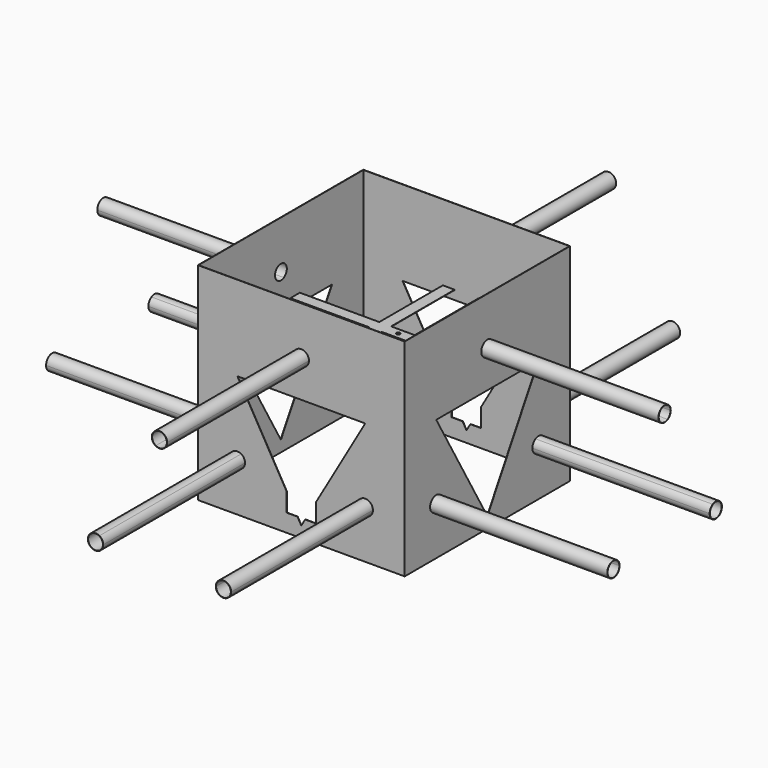
from build123d import *

# Parameters (mm, degrees)
F0_W      = 700
F0_H      = 700
F0_W_2    = 698
F0_H_2    = 698
F1_DEPTH  = 700
F6_DEPTH  = 600
F7_DEPTH  = 600
F8_DEPTH  = 600
F9_DEPTH  = 600
F10_DEPTH = 25
F11_DEPTH = 25
F12_DEPTH = 25
F13_DEPTH = 25
F14_DEPTH = 25
F15_DEPTH = 25
F16_DEPTH = 4990
F17_DEPTH = 700
F18_DEPTH = 700
F19_DEPTH = 700
F20_DEPTH = 700
F21_W     = 100
F21_H     = 80
F22_DEPTH = 350
F24_D     = 13
F24_DEPTH = 5
F24_TIP   = 3.905594


with BuildPart() as f1:
    # F0 (on Top) → F1 (new body)
    with BuildSketch(Plane.XY):
        Rectangle(F0_W, F0_H)
        Rectangle(F0_W_2, F0_H_2, mode=Mode.SUBTRACT)
    extrude(amount=-F1_DEPTH)

    # F2 (on face) → F6 (join)
    with BuildSketch(Plane.YZ.offset(350)):
        with BuildLine():
            ThreePointArc((25, -162.5), (21.650635, -175), (12.5, -184.150635))
            Line((12.5, -184.150635), (13, -185.01666))
            ThreePointArc((13, -185.01666), (22.51666, -175.5), (26, -162.5))
            ThreePointArc((26, -162.5), (-13, -139.98334), (-13, -185.01666))
            Line((-13, -185.01666), (-12.5, -184.150635))
            ThreePointArc((-12.5, -184.150635), (-12.5, -140.849365), (25, -162.5))
        make_face()
        with BuildLine():
            ThreePointArc((242.506351, -537.5), (229.506351, -514.98334), (203.506351, -514.98334))
            Line((203.506351, -514.98334), (204.006351, -515.849365))
            ThreePointArc((204.006351, -515.849365), (229.006351, -515.849365), (241.506351, -537.5))
            ThreePointArc((241.506351, -537.5), (216.506351, -562.5), (191.506351, -537.5))
            Line((191.506351, -537.5), (190.506351, -537.5))
            ThreePointArc((190.506351, -537.5), (216.506351, -563.5), (242.506351, -537.5))
        make_face()
        with BuildLine():
            Line((204.006351, -515.849365), (203.506351, -514.98334))
            ThreePointArc((203.506351, -514.98334), (193.98969, -524.5), (190.506351, -537.5))
            Line((190.506351, -537.5), (191.506351, -537.5))
            ThreePointArc((191.506351, -537.5), (194.855716, -525), (204.006351, -515.849365))
        make_face()
        with BuildLine():
            Line((13, -185.01666), (12.5, -184.150635))
            ThreePointArc((12.5, -184.150635), (0, -187.5), (-12.5, -184.150635))
            Line((-12.5, -184.150635), (-13, -185.01666))
            ThreePointArc((-13, -185.01666), (0, -188.5), (13, -185.01666))
        make_face()
        with BuildLine():
            Line((-204.006351, -515.849365), (-203.506351, -514.98334))
            ThreePointArc((-203.506351, -514.98334), (-239.023011, -550.5), (-190.506351, -537.5))
            Line((-190.506351, -537.5), (-191.506351, -537.5))
            ThreePointArc((-191.506351, -537.5), (-238.156986, -550), (-204.006351, -515.849365))
        make_face()
        with BuildLine():
            ThreePointArc((-190.506351, -537.5), (-193.98969, -524.5), (-203.506351, -514.98334))
            Line((-203.506351, -514.98334), (-204.006351, -515.849365))
            ThreePointArc((-204.006351, -515.849365), (-194.855716, -525), (-191.506351, -537.5))
            Line((-191.506351, -537.5), (-190.506351, -537.5))
        make_face()
    extrude(amount=F6_DEPTH)

    # F3 (on face) → F7 (join)
    with BuildSketch(Plane.XZ.offset(350)):
        with BuildLine():
            Line((13, -185.01666), (12.5, -184.150635))
            ThreePointArc((12.5, -184.150635), (0, -187.5), (-12.5, -184.150635))
            Line((-12.5, -184.150635), (-13, -185.01666))
            ThreePointArc((-13, -185.01666), (0, -188.5), (13, -185.01666))
        make_face()
        with BuildLine():
            ThreePointArc((25, -162.5), (21.650635, -175), (12.5, -184.150635))
            Line((12.5, -184.150635), (13, -185.01666))
            ThreePointArc((13, -185.01666), (22.51666, -175.5), (26, -162.5))
            ThreePointArc((26, -162.5), (-13, -139.98334), (-13, -185.01666))
            Line((-13, -185.01666), (-12.5, -184.150635))
            ThreePointArc((-12.5, -184.150635), (-12.5, -140.849365), (25, -162.5))
        make_face()
        with BuildLine():
            Line((-204.006351, -515.849365), (-203.506351, -514.98334))
            ThreePointArc((-203.506351, -514.98334), (-239.023011, -550.5), (-190.506351, -537.5))
            Line((-190.506351, -537.5), (-191.506351, -537.5))
            ThreePointArc((-191.506351, -537.5), (-238.156986, -550), (-204.006351, -515.849365))
        make_face()
        with BuildLine():
            ThreePointArc((-190.506351, -537.5), (-193.98969, -524.5), (-203.506351, -514.98334))
            Line((-203.506351, -514.98334), (-204.006351, -515.849365))
            ThreePointArc((-204.006351, -515.849365), (-194.855716, -525), (-191.506351, -537.5))
            Line((-191.506351, -537.5), (-190.506351, -537.5))
        make_face()
        with BuildLine():
            ThreePointArc((242.506351, -537.5), (229.506351, -514.98334), (203.506351, -514.98334))
            Line((203.506351, -514.98334), (204.006351, -515.849365))
            ThreePointArc((204.006351, -515.849365), (229.006351, -515.849365), (241.506351, -537.5))
            ThreePointArc((241.506351, -537.5), (216.506351, -562.5), (191.506351, -537.5))
            Line((191.506351, -537.5), (190.506351, -537.5))
            ThreePointArc((190.506351, -537.5), (216.506351, -563.5), (242.506351, -537.5))
        make_face()
        with BuildLine():
            Line((204.006351, -515.849365), (203.506351, -514.98334))
            ThreePointArc((203.506351, -514.98334), (193.98969, -524.5), (190.506351, -537.5))
            Line((190.506351, -537.5), (191.506351, -537.5))
            ThreePointArc((191.506351, -537.5), (194.855716, -525), (204.006351, -515.849365))
        make_face()
    extrude(amount=F7_DEPTH)

    # F4 (on face) → F8 (join)
    with BuildSketch(Plane(origin=(-350, 0, 0), x_dir=(0, -1, 0), z_dir=(-1, 0, 0))):
        with BuildLine():
            ThreePointArc((25, -162.5), (21.650635, -175), (12.5, -184.150635))
            Line((12.5, -184.150635), (13, -185.01666))
            ThreePointArc((13, -185.01666), (22.51666, -175.5), (26, -162.5))
            ThreePointArc((26, -162.5), (-13, -139.98334), (-13, -185.01666))
            Line((-13, -185.01666), (-12.5, -184.150635))
            ThreePointArc((-12.5, -184.150635), (-12.5, -140.849365), (25, -162.5))
        make_face()
        with BuildLine():
            Line((13, -185.01666), (12.5, -184.150635))
            ThreePointArc((12.5, -184.150635), (0, -187.5), (-12.5, -184.150635))
            Line((-12.5, -184.150635), (-13, -185.01666))
            ThreePointArc((-13, -185.01666), (0, -188.5), (13, -185.01666))
        make_face()
        with BuildLine():
            ThreePointArc((242.506351, -537.5), (229.506351, -514.98334), (203.506351, -514.98334))
            Line((203.506351, -514.98334), (204.006351, -515.849365))
            ThreePointArc((204.006351, -515.849365), (229.006351, -515.849365), (241.506351, -537.5))
            ThreePointArc((241.506351, -537.5), (216.506351, -562.5), (191.506351, -537.5))
            Line((191.506351, -537.5), (190.506351, -537.5))
            ThreePointArc((190.506351, -537.5), (216.506351, -563.5), (242.506351, -537.5))
        make_face()
        with BuildLine():
            Line((204.006351, -515.849365), (203.506351, -514.98334))
            ThreePointArc((203.506351, -514.98334), (193.98969, -524.5), (190.506351, -537.5))
            Line((190.506351, -537.5), (191.506351, -537.5))
            ThreePointArc((191.506351, -537.5), (194.855716, -525), (204.006351, -515.849365))
        make_face()
        with BuildLine():
            Line((-204.006351, -515.849365), (-203.506351, -514.98334))
            ThreePointArc((-203.506351, -514.98334), (-239.023011, -550.5), (-190.506351, -537.5))
            Line((-190.506351, -537.5), (-191.506351, -537.5))
            ThreePointArc((-191.506351, -537.5), (-238.156986, -550), (-204.006351, -515.849365))
        make_face()
        with BuildLine():
            ThreePointArc((-190.506351, -537.5), (-193.98969, -524.5), (-203.506351, -514.98334))
            Line((-203.506351, -514.98334), (-204.006351, -515.849365))
            ThreePointArc((-204.006351, -515.849365), (-194.855716, -525), (-191.506351, -537.5))
            Line((-191.506351, -537.5), (-190.506351, -537.5))
        make_face()
    extrude(amount=F8_DEPTH)

    # F5 (on face) → F9 (join)
    with BuildSketch(Plane(origin=(0, 350, 0), x_dir=(-1, 0, 0), z_dir=(0, 1, 0))):
        with BuildLine():
            Line((13, -185.01666), (12.5, -184.150635))
            ThreePointArc((12.5, -184.150635), (0, -187.5), (-12.5, -184.150635))
            Line((-12.5, -184.150635), (-13, -185.01666))
            ThreePointArc((-13, -185.01666), (0, -188.5), (13, -185.01666))
        make_face()
        with BuildLine():
            ThreePointArc((25, -162.5), (21.650635, -175), (12.5, -184.150635))
            Line((12.5, -184.150635), (13, -185.01666))
            ThreePointArc((13, -185.01666), (22.51666, -175.5), (26, -162.5))
            ThreePointArc((26, -162.5), (-13, -139.98334), (-13, -185.01666))
            Line((-13, -185.01666), (-12.5, -184.150635))
            ThreePointArc((-12.5, -184.150635), (-12.5, -140.849365), (25, -162.5))
        make_face()
        with BuildLine():
            Line((-204.006351, -515.849365), (-203.506351, -514.98334))
            ThreePointArc((-203.506351, -514.98334), (-239.023011, -550.5), (-190.506351, -537.5))
            Line((-190.506351, -537.5), (-191.506351, -537.5))
            ThreePointArc((-191.506351, -537.5), (-238.156986, -550), (-204.006351, -515.849365))
        make_face()
        with BuildLine():
            ThreePointArc((-190.506351, -537.5), (-193.98969, -524.5), (-203.506351, -514.98334))
            Line((-203.506351, -514.98334), (-204.006351, -515.849365))
            ThreePointArc((-204.006351, -515.849365), (-194.855716, -525), (-191.506351, -537.5))
            Line((-191.506351, -537.5), (-190.506351, -537.5))
        make_face()
        with BuildLine():
            Line((204.006351, -515.849365), (203.506351, -514.98334))
            ThreePointArc((203.506351, -514.98334), (193.98969, -524.5), (190.506351, -537.5))
            Line((190.506351, -537.5), (191.506351, -537.5))
            ThreePointArc((191.506351, -537.5), (194.855716, -525), (204.006351, -515.849365))
        make_face()
        with BuildLine():
            ThreePointArc((242.506351, -537.5), (229.506351, -514.98334), (203.506351, -514.98334))
            Line((203.506351, -514.98334), (204.006351, -515.849365))
            ThreePointArc((204.006351, -515.849365), (229.006351, -515.849365), (241.506351, -537.5))
            ThreePointArc((241.506351, -537.5), (216.506351, -562.5), (191.506351, -537.5))
            Line((191.506351, -537.5), (190.506351, -537.5))
            ThreePointArc((190.506351, -537.5), (216.506351, -563.5), (242.506351, -537.5))
        make_face()
    extrude(amount=F9_DEPTH)

    # F10 (cut): a face of the model
    f10_faces = [f1.faces().sort_by_distance(p)[0] for p in [
        (350, -216.506351, -537.5),
    ]]
    extrude(f10_faces, amount=-F10_DEPTH, mode=Mode.SUBTRACT)

    # F11 (cut): a face of the model
    f11_faces = [f1.faces().sort_by_distance(p)[0] for p in [
        (350, 216.506351, -537.5),
    ]]
    extrude(f11_faces, amount=-F11_DEPTH, mode=Mode.SUBTRACT)

    # F12 (cut): a face of the model
    f12_faces = [f1.faces().sort_by_distance(p)[0] for p in [
        (-350, 216.506351, -537.5),
    ]]
    extrude(f12_faces, amount=-F12_DEPTH, mode=Mode.SUBTRACT)

    # F13 (cut): a face of the model
    f13_faces = [f1.faces().sort_by_distance(p)[0] for p in [
        (-350, -216.506351, -537.5),
    ]]
    extrude(f13_faces, amount=-F13_DEPTH, mode=Mode.SUBTRACT)

    # F14 (cut): faces of the model
    f14_faces = [f1.faces().sort_by_distance(p)[0] for p in [
        (-216.506351, 350, -537.5),
        (216.506351, 350, -537.5),
    ]]
    extrude(f14_faces, amount=-F14_DEPTH, mode=Mode.SUBTRACT)

    # F15 (cut): faces of the model
    f15_faces = [f1.faces().sort_by_distance(p)[0] for p in [
        (216.506351, -350, -537.5),
        (-216.506351, -350, -537.5),
    ]]
    extrude(f15_faces, amount=-F15_DEPTH, mode=Mode.SUBTRACT)

    # F16 (cut): a face of the model
    f16_faces = [f1.faces().sort_by_distance(p)[0] for p in [
        (350, 0, -162.5),
    ]]
    extrude(f16_faces, amount=-F16_DEPTH, mode=Mode.SUBTRACT)

    # F2 (on face) → F17 (cut)
    with BuildSketch(Plane.YZ.offset(350)):
        Polygon((216.506351, -287.5), (72.168784, -287.5), (144.337567, -412.5), align=None)
        Polygon((144.337567, -412.5), (72.168784, -287.5), (-72.168784, -287.5), (-144.337567, -412.5), (-72.168784, -537.5), (72.168784, -537.5), align=None)
        Polygon((-144.337567, -412.5), (-72.168784, -287.5), (-216.506351, -287.5), align=None)
        Polygon((0, -662.5), (72.168784, -537.5), (-72.168784, -537.5), align=None)
    extrude(amount=-F17_DEPTH, mode=Mode.SUBTRACT)

    # F3 (on face) → F18 (cut)
    with BuildSketch(Plane.XZ.offset(350)):
        Polygon((-144.337567, -412.5), (-72.168784, -287.5), (-216.506351, -287.5), align=None)
        Polygon((144.337567, -412.5), (72.168784, -287.5), (-72.168784, -287.5), (-144.337567, -412.5), (-72.168784, -537.5), (72.168784, -537.5), align=None)
        Polygon((216.506351, -287.5), (72.168784, -287.5), (144.337567, -412.5), align=None)
        Polygon((0, -662.5), (72.168784, -537.5), (-72.168784, -537.5), align=None)
    extrude(amount=-F18_DEPTH, mode=Mode.SUBTRACT)

    # F2 (on face) → F19 (join)
    with BuildSketch(Plane.YZ.offset(350)):
        Polygon((-54.848276, -257.5), (-54.270925, -256.5), (-80, -256.5), (-80, -257.5), align=None)
        Polygon((-40, -256.5), (-54.270925, -256.5), (-54.848276, -257.5), (-40, -257.5), align=None)
        Polygon((54.848276, -257.5), (54.270925, -256.5), (40, -256.5), (40, -257.5), align=None)
        Polygon((80, -256.5), (54.270925, -256.5), (54.848276, -257.5), (80, -257.5), align=None)
    extrude(amount=-F19_DEPTH)

    # F3 (on face) → F20 (join)
    with BuildSketch(Plane.XZ.offset(350)):
        Polygon((-54.848276, -257.5), (-54.270925, -256.5), (-80, -256.5), (-80, -257.5), align=None)
        Polygon((-40, -256.5), (-54.270925, -256.5), (-54.848276, -257.5), (-40, -257.5), align=None)
        Polygon((54.848276, -257.5), (54.270925, -256.5), (40, -256.5), (40, -257.5), align=None)
        Polygon((80, -256.5), (54.270925, -256.5), (54.848276, -257.5), (80, -257.5), align=None)
    extrude(amount=-F20_DEPTH)

    # F21 (on Front) → F22 (cut, symmetric)
    with BuildSketch(Plane.XZ):
        with Locations((0, -600)):
            Rectangle(F21_W, F21_H)
    extrude(amount=F22_DEPTH, both=True, mode=Mode.SUBTRACT)

    # F24
    with Locations(Plane.XY.offset(-256.5)):
        with Locations((0, 60), (-60, 0), (0, -60), (60, 0)):
            Hole(F24_D / 2, depth=F24_DEPTH)
            with Locations((0, 0, -(F24_DEPTH + F24_TIP / 2))):  # 118° drill point
                Cone(0, F24_D / 2, F24_TIP, mode=Mode.SUBTRACT)


solid = f1.part
